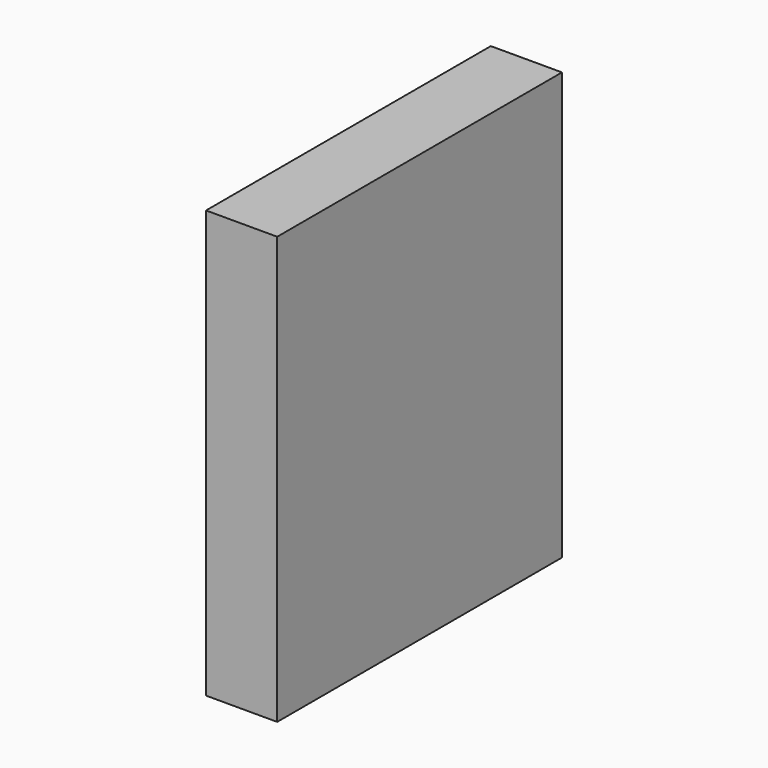
from build123d import *

# Parameters (mm, degrees)
F0_W     = 6.35
F0_H     = 38.1
F1_DEPTH = 31.75
F2_W     = 5.4897969239
F2_H     = 1.5875
F2_W_2   = 5.5069834925
F3_DEPTH = 0.396875


# Not quite as in the source:
# - a length typed as a fraction of an inch, garbled in the dataset ("3 / 203.2 mm" for 3/8 in), is restored


with BuildPart() as f1:
    # F0 (on Front) → F1 (new body)
    with BuildSketch(Plane.XZ):
        Rectangle(F0_W, F0_H)
    extrude(amount=F1_DEPTH)

    # F2 (on Front) → F3 (cut)
    with BuildSketch(Plane.XZ):
        with Locations((0.0038447615, -2.38125)):
            Rectangle(F2_W, F2_H)
        with Locations((0.0038447615, -4.365625)):
            Rectangle(F2_W, F2_H)
        with Locations((-0.0047485228, -6.35)):
            Rectangle(F2_W_2, F2_H)
    extrude(amount=F3_DEPTH, mode=Mode.SUBTRACT)


solid = f1.part
